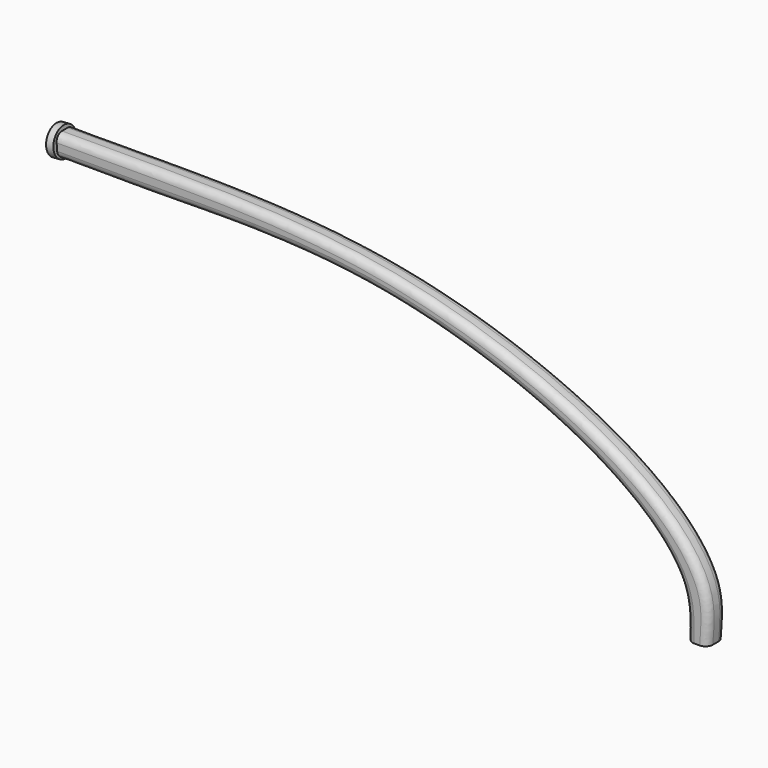
from build123d import *

# Parameters (mm, degrees)
F1_DEPTH = 3
F2_R     = 1
F3_R     = 1.9834594101
F4_DEPTH = 1


with BuildPart() as f1:
    # F0 (on Front) → F1 (new body)
    with BuildSketch(Plane.XZ):
        with BuildLine():
            add(Edge.make_bspline(
                [(-60.1259171963, 26.6715344042), (-45.950281109, 26.5863429632), (-16.1966218447, 27.9811763069), (19.7828472581, 13.3653801763), (30.2059783266, 0.9370018135), (29.4527750191, -4.5178706528), (29.3156970292, -6.4025372267)],
                knots=[0, 0, 0, 0, 0.3490384499, 0.6710290853, 0.8677913228, 1, 1, 1, 1], degree=3))
            Line((-60.1259171963, 26.6715344042), (-59.8959885538, 23.6824825406))
            add(Edge.make_bspline(
                [(-59.8959885538, 23.6824825406), (-55.7242948882, 23.7491967997), (-45.9801272737, 23.4902373676), (-16.3011036479, 24.5030395159), (14.7814330999, 12.9920368732), (27.067114625, 1.1147458899), (26.5215866088, -4.5454404746), (26.5565682203, -6.4025372267)],
                knots=[0, 0, 0, 0, 0.1708389276, 0.4257579814, 0.6983991748, 0.8812846646, 1, 1, 1, 1], degree=3))
            Line((26.5565682203, -6.4025372267), (29.3156970292, -6.4025372267))
        make_face()
    extrude(amount=F1_DEPTH)

    # F2
    f2_edges = [f1.edges().sort_by_distance(p)[0] for p in [
        (-8.468397, -3, 23.066336),
        (-8.468397, 0, 23.066336),
        (-10.479506, 0, 21.01023),
        (-10.479506, -3, 21.01023),
    ]]
    fillet(f2_edges, radius=F2_R)

    # F3 (on face) → F4 (join)
    with BuildSketch(Plane(origin=(-57.7326287688, 0, -4.4410018853), x_dir=(0, -1, 0), z_dir=(-0.9970544453, 0, -0.0766970215))):
        with Locations((1.6133522149, 29.791906476)):
            Circle(F3_R)
    extrude(amount=F4_DEPTH)


solid = f1.part
